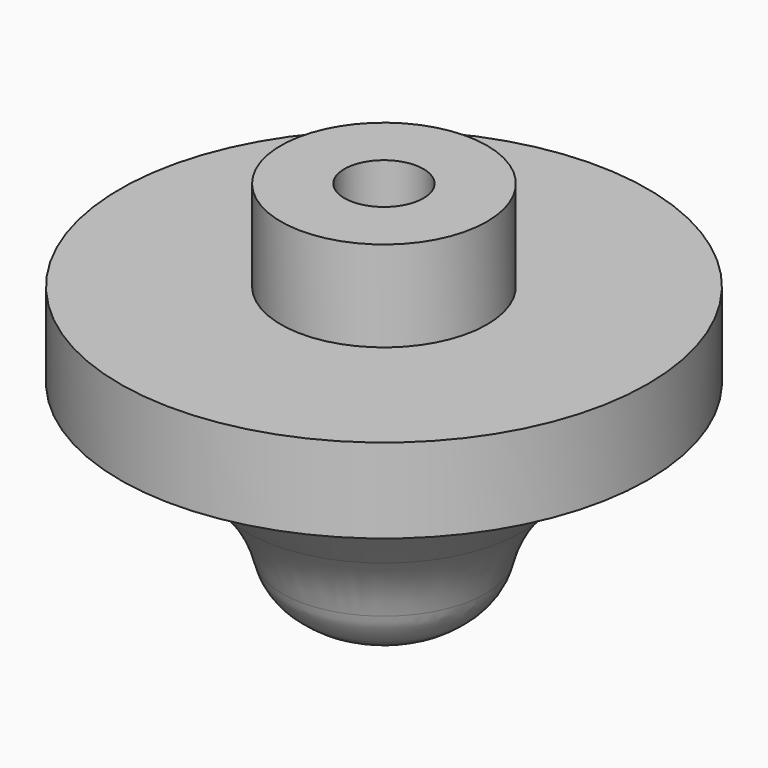
from build123d import *

# Parameters (mm, degrees)
F2_R     = 4.7625
F3_DEPTH = 24.765
F4_R     = 1.5875
F5_DEPTH = 9.525
F7_R     = 7.62


# Not quite as in the source:
# - a fillet or chamfer that OpenCascade refuses, or shapes differently, is made with other operations: its cross-section is extruded or revolved along the edge and cut away or added


with BuildPart() as f1:
    # F0 (on Front) → F1 (revolve)
    with BuildSketch(Plane.XZ):
        Polygon((11.8329105899, 9.1992265151), (26.5666254177, 24.660434838), (31.75, 24.660434838), (31.75, 34.820434838), (12.3952, 34.820434838), (12.3952, 45.72), (0, 45.72), (0, 0), (4.4022302061, 0), (9.0794198883, 6.3097791593), align=None)
        Polygon((11.8329105899, 3.9054930676), (11.8329105899, 9.1992265151), (9.0794198883, 6.3097791593), (4.4022302061, 0), (6.9125830196, 0), align=None)
    revolve(axis=Axis((0, 0, 22.86), (0, 0, -1)))

    # F2 (on face) → F3 (cut)
    with BuildSketch(Plane.XY.offset(45.72)):
        Circle(F2_R)
    extrude(amount=-F3_DEPTH, mode=Mode.SUBTRACT)

    # F4 (on face) → F5 (cut)
    with BuildSketch(Plane(origin=(0, 0, 0), x_dir=(1, 0, 0), z_dir=(0, 0, -1))):
        Circle(F4_R)
    extrude(amount=-F5_DEPTH, mode=Mode.SUBTRACT)

    # F6: fillet of radius 17.3381993495 on 3 edges, made by hand

    # F6_s1 → F6_t2 (revolve)
    with BuildSketch(Plane.XZ):
        with BuildLine():
            ThreePointArc((16.5322882716, 14.130641177), (13.3299473179, 9.4099376621), (11.8329105899, 3.9054930676))
            Line((11.8329105899, 3.9054930676), (11.4878890775, 3.9402122077))
            ThreePointArc((11.4878890775, 3.9402122077), (11.4861466029, 6.5523597914), (11.4861466029, 9.1992265151))
            Line((11.4861466029, 9.1992265151), (11.5818766312, 9.4384486175))
            Line((11.5818766312, 9.4384486175), (16.2812543129, 14.3698632794))
            Line((16.2812543129, 14.3698632794), (16.5322882716, 14.130641177))
        make_face()
    revolve(axis=Axis((0, 0, 9.1992265151), (0, 0, -1)))

    # F6_s3 → F6_t4 (revolve)
    with BuildSketch(Plane.XZ):
        with BuildLine():
            ThreePointArc((21.6021022057, 19.4507827916), (26.2353502113, 22.9140514833), (31.75, 24.660434838))
            Line((31.75, 24.660434838), (31.7019239972, 25.0038499813))
            ThreePointArc((31.7019239972, 25.0038499813), (29.1583127088, 25.007198825), (26.5666254177, 25.007198825))
            Line((26.5666254177, 25.007198825), (26.3155914589, 24.8996569403))
            Line((26.3155914589, 24.8996569403), (21.351068247, 19.6900048939))
            Line((21.351068247, 19.6900048939), (21.6021022057, 19.4507827916))
        make_face()
    revolve(axis=Axis((0, 0, 24.660434838), (0, 0, -1)))

    # F7
    f7_edges = [f1.edges().sort_by_distance(p)[0] for p in [
        (9.372747, 0, 1.952747),
        (-11.832911, 0, 3.905493),
        (-6.912583, 0, 0),
    ]]
    fillet(f7_edges, radius=F7_R)


solid = f1.part
